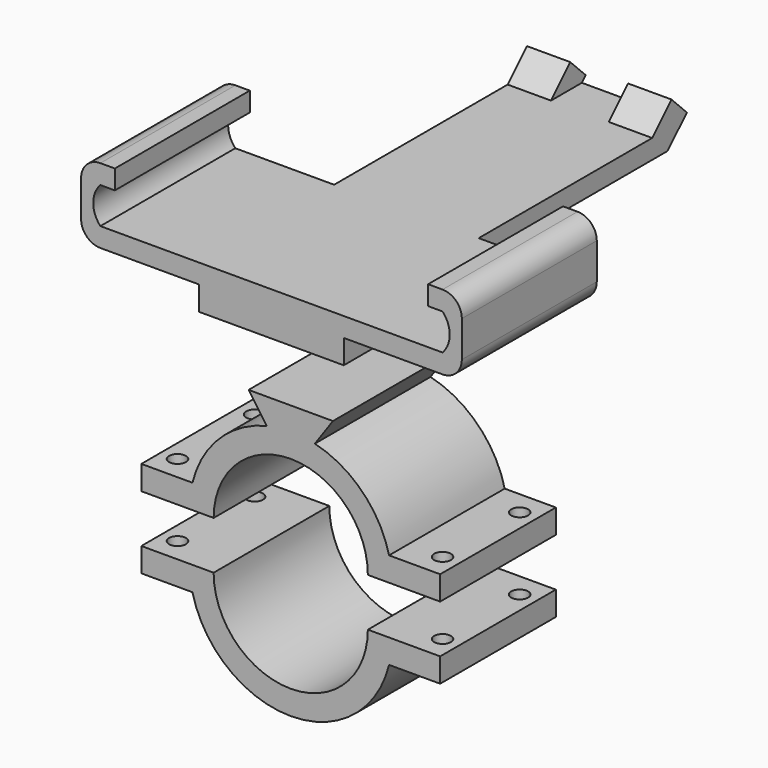
from build123d import *

# Parameters (mm, degrees)
F3_DEPTH      = 30
F4_DEPTH      = 5
F6_DEPTH      = 15
F6_DEPTH_BACK = 15
F7_DEPTH      = 6
F8_DEPTH      = 30
F9_DEPTH      = 30
F10_R         = 1.75
F11_DEPTH     = 50


# Not quite as in the source:
# - a feature names something its author has since deleted; it is built from what else it names


with BuildPart() as f3:
    # F2 (on offset) → F3 (new body)
    with BuildSketch(Plane.XZ.offset(30)):
        with BuildLine():
            Line((35.5, 49), (-35.5, 49))
            ThreePointArc((-35.5, 49), (-36.9829280499, 52.75), (-35.5, 56.5))
            Line((-35.5, 56.5), (-32.5, 56.5))
            Line((-32.5, 56.5), (-32.5, 60.5))
            Line((-32.5, 60.5), (-35.5, 60.5))
            ThreePointArc((-35.5, 60.5), (-38.3284271247, 59.3284271247), (-39.5, 56.5))
            Line((-39.5, 56.5), (-39.5, 49))
            ThreePointArc((-39.5, 49), (-38.3284271247, 46.1715728753), (-35.5, 45))
            Line((-35.5, 45), (-15, 45))
            Line((-15, 45), (-15, 40))
            Line((-15, 40), (-5.798962309, 40))
            Line((-5.798962309, 40), (-9.3, 45))
            Line((-9.3, 45), (9.3, 45))
            Line((9.3, 45), (5.798962309, 40))
            Line((5.798962309, 40), (15, 40))
            Line((15, 40), (15, 45))
            Line((15, 45), (35.5, 45))
            ThreePointArc((35.5, 45), (38.3284271247, 46.1715728753), (39.5, 49))
            Line((39.5, 49), (39.5, 56.5))
            ThreePointArc((39.5, 56.5), (38.3284271247, 59.3284271247), (35.5, 60.5))
            Line((35.5, 60.5), (32.5, 60.5))
            Line((32.5, 60.5), (32.5, 56.5))
            Line((32.5, 56.5), (35.5, 56.5))
            ThreePointArc((35.5, 56.5), (36.9829280499, 52.75), (35.5, 49))
        make_face()
    extrude(amount=-F3_DEPTH)

    # F2 (on offset) → F4 (join)
    with BuildSketch(Plane.XZ.offset(30)):
        with BuildLine():
            Line((35.5, 49), (-35.5, 49))
            ThreePointArc((-35.5, 49), (-36.9829280499, 52.75), (-35.5, 56.5))
            Line((-35.5, 56.5), (-32.5, 56.5))
            Line((-32.5, 56.5), (-32.5, 60.5))
            Line((-32.5, 60.5), (-35.5, 60.5))
            ThreePointArc((-35.5, 60.5), (-38.3284271247, 59.3284271247), (-39.5, 56.5))
            Line((-39.5, 56.5), (-39.5, 49))
            ThreePointArc((-39.5, 49), (-38.3284271247, 46.1715728753), (-35.5, 45))
            Line((-35.5, 45), (-15, 45))
            Line((-15, 45), (-15, 40))
            Line((-15, 40), (-5.798962309, 40))
            Line((-5.798962309, 40), (-9.3, 45))
            Line((-9.3, 45), (9.3, 45))
            Line((9.3, 45), (5.798962309, 40))
            Line((5.798962309, 40), (15, 40))
            Line((15, 40), (15, 45))
            Line((15, 45), (35.5, 45))
            ThreePointArc((35.5, 45), (38.3284271247, 46.1715728753), (39.5, 49))
            Line((39.5, 49), (39.5, 56.5))
            ThreePointArc((39.5, 56.5), (38.3284271247, 59.3284271247), (35.5, 60.5))
            Line((35.5, 60.5), (32.5, 60.5))
            Line((32.5, 60.5), (32.5, 56.5))
            Line((32.5, 56.5), (35.5, 56.5))
            ThreePointArc((35.5, 56.5), (36.9829280499, 52.75), (35.5, 49))
        make_face()
        Polygon((-9.3, 45), (-5.798962309, 40), (5.798962309, 40), (9.3, 45), align=None)
    extrude(amount=F4_DEPTH)

    # F5 (on Right) → F6 (join, two sides)
    with BuildSketch(Plane.YZ) as f6_sk:
        Polygon((45, 49), (0, 49), (0, 45), (49, 45), (53, 49), align=None)
        Polygon((50, 54), (45, 49), (53, 49), (54, 50), align=None)
    extrude(amount=F6_DEPTH)
    extrude(f6_sk.sketch, amount=-F6_DEPTH_BACK)

    # F5 (on Right) → F7 (cut, symmetric)
    with BuildSketch(Plane.YZ):
        Polygon((50, 54), (45, 49), (53, 49), (54, 50), align=None)
    extrude(amount=F7_DEPTH, both=True, mode=Mode.SUBTRACT)


with BuildPart() as f8:
    # F0 (on Front) → F8 (new body)
    with BuildSketch(Plane.XZ):
        with BuildLine():
            Line((-31, 0), (-21, 0))
            ThreePointArc((-21, 0), (-20.8484728355, 2.5181700556), (-20.3960780544, 5))
            Line((-20.3960780544, 5), (-31, 5))
            Line((-31, 5), (-31, 0))
        make_face()
        with BuildLine():
            Line((-21, 0), (-16, 0))
            Line((-16, 0), (-16, 5))
            Line((-16, 5), (-20.3960780544, 5))
            ThreePointArc((-20.3960780544, 5), (-20.8484728355, 2.5181700556), (-21, 0))
        make_face()
        with BuildLine():
            ThreePointArc((-16, 0), (0, 16), (16, 0))
            Line((16, 0), (16, 5))
            Line((16, 5), (20.3960780544, 5))
            ThreePointArc((20.3960780544, 5), (14.8492424049, 14.8492424049), (5, 20.3960780544))
            ThreePointArc((5, 20.3960780544), (0, 21), (-5, 20.3960780544))
            ThreePointArc((-5, 20.3960780544), (-14.8492424049, 14.8492424049), (-20.3960780544, 5))
            Line((-20.3960780544, 5), (-16, 5))
            Line((-16, 5), (-16, 0))
        make_face()
        with BuildLine():
            Line((16, 5), (16, 0))
            Line((16, 0), (21, 0))
            ThreePointArc((21, 0), (20.8484728355, 2.5181700556), (20.3960780544, 5))
            Line((20.3960780544, 5), (16, 5))
        make_face()
        with BuildLine():
            ThreePointArc((20.3960780544, 5), (20.8484728355, 2.5181700556), (21, 0))
            Line((21, 0), (31, 0))
            Line((31, 0), (31, 5))
            Line((31, 5), (20.3960780544, 5))
        make_face()
        with BuildLine():
            ThreePointArc((-5, 20.3960780544), (0, 21), (5, 20.3960780544))
            Line((5, 20.3960780544), (8.75, 25.7516330797))
            Line((8.75, 25.7516330797), (-8.75, 25.7516330797))
            Line((-8.75, 25.7516330797), (-5, 20.3960780544))
        make_face()
    extrude(amount=F8_DEPTH)


with BuildPart() as f9:
    # F0 (on Front) → F9 (new body)
    with BuildSketch(Plane.XZ):
        with BuildLine():
            ThreePointArc((-20.3960780544, -15), (-20.8484728355, -12.5181700556), (-21, -10))
            Line((-21, -10), (-31, -10))
            Line((-31, -10), (-31, -15))
            Line((-31, -15), (-20.3960780544, -15))
        make_face()
        with BuildLine():
            Line((-16, -15), (-16, -10))
            Line((-16, -10), (-21, -10))
            ThreePointArc((-21, -10), (-20.8484728355, -12.5181700556), (-20.3960780544, -15))
            Line((-20.3960780544, -15), (-16, -15))
        make_face()
        with BuildLine():
            ThreePointArc((16, -10), (0, -26), (-16, -10))
            Line((-16, -10), (-16, -15))
            Line((-16, -15), (-20.3960780544, -15))
            ThreePointArc((-20.3960780544, -15), (0, -31), (20.3960780544, -15))
            Line((20.3960780544, -15), (16, -15))
            Line((16, -15), (16, -10))
        make_face()
        with BuildLine():
            Line((21, -10), (16, -10))
            Line((16, -10), (16, -15))
            Line((16, -15), (20.3960780544, -15))
            ThreePointArc((20.3960780544, -15), (20.8484728355, -12.5181700556), (21, -10))
        make_face()
        with BuildLine():
            Line((31, -10), (21, -10))
            ThreePointArc((21, -10), (20.8484728355, -12.5181700556), (20.3960780544, -15))
            Line((20.3960780544, -15), (31, -15))
            Line((31, -15), (31, -10))
        make_face()
    extrude(amount=F9_DEPTH)


with BuildPart() as f11_tool:
    # F10 (on face) → F11 (new body)
    with BuildSketch(Plane.XY.offset(5)):
        with Locations((-27.5, -25)):
            Circle(F10_R)
        with Locations((-27.5, -5)):
            Circle(F10_R)
        with Locations((27.5, -5)):
            Circle(F10_R)
        with Locations((27.5, -25)):
            Circle(F10_R)
    extrude(amount=-F11_DEPTH)


with BuildPart() as f8_1:
    add(f8.part)

    # F11: cut by f11_tool
    add(f11_tool.part, mode=Mode.SUBTRACT)


with BuildPart() as f9_1:
    add(f9.part)

    # F11: cut by f11_tool
    add(f11_tool.part, mode=Mode.SUBTRACT)


solid = Compound([f3.part, f8_1.part, f9_1.part])
